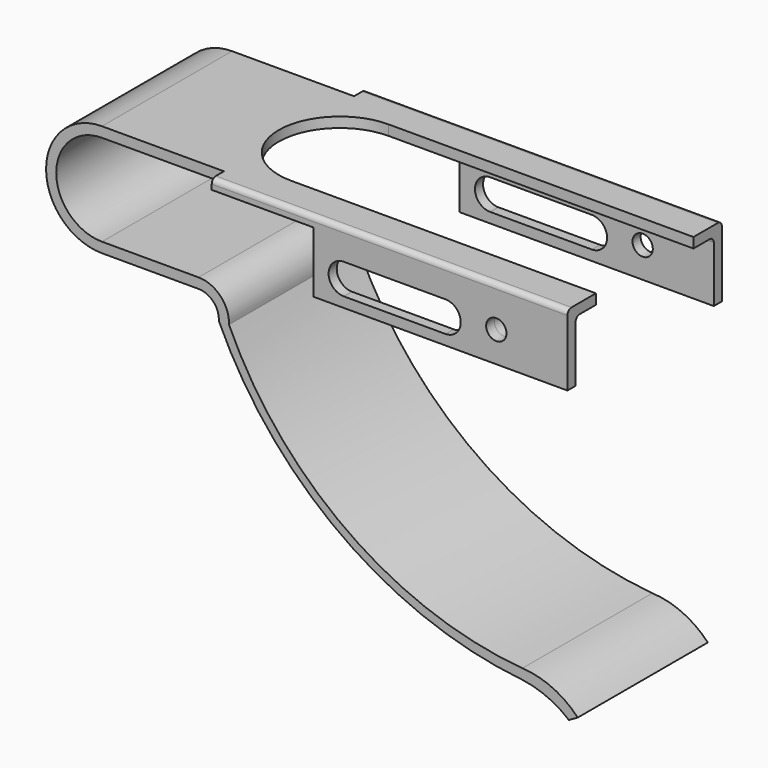
from build123d import *

# Parameters (mm, degrees)
F1_DEPTH  = 16
F2_W      = 70
F2_H      = 3
F3_DEPTH  = 2
F4_W      = 50
F4_H      = 12
F5_DEPTH  = 2
F6_R      = 1
F9_DEPTH  = 2
F11_DEPTH = 38.001
F13_D     = 4
F14_R     = 3
F14_R_2   = 2
F15_DEPTH = 5


with BuildPart() as f1:
    # F0 (on Front) → F1 (new body)
    with BuildSketch(Plane.XZ):
        with BuildLine():
            Line((46.2855722755, 5.7414249778), (-47.7144277245, 5.7414249778))
            ThreePointArc((-47.7144277245, 5.7414249778), (-58.7144277245, -5.2585750222), (-47.7144277245, -16.2585750222))
            Line((-47.7144277245, -16.2585750222), (-28.7144277245, -16.2585750222))
            ThreePointArc((-28.7144277245, -16.2585750222), (-25.7968307423, -17.5210599177), (-24.7197856057, -20.5120821569))
            ThreePointArc((-24.7197856057, -20.5120821569), (-0.5386319719, -49.8206199667), (35.0020481502, -63.2585750222))
            ThreePointArc((35.0020481502, -63.2585750222), (39.8678360266, -64.6074545818), (44.1721712505, -67.2471640366))
            Line((44.1721712505, -67.2471640366), (45.9107602648, -66.2585750222))
            ThreePointArc((45.9107602648, -66.2585750222), (40.9429054682, -62.6971545828), (35.0020481502, -61.2585750222))
            ThreePointArc((35.0020481502, -61.2585750222), (0.6230450398, -48.7022972109), (-22.7197856057, -20.5120821569))
            ThreePointArc((-22.7197856057, -20.5120821569), (-24.3830859689, -16.1065299122), (-28.7144277245, -14.2585750222))
            Line((-28.7144277245, -14.2585750222), (-47.7144277245, -14.2585750222))
            ThreePointArc((-47.7144277245, -14.2585750222), (-56.7144277245, -5.2585750222), (-47.7144277245, 3.7414249778))
            Line((-47.7144277245, 3.7414249778), (46.2855722755, 3.7414249778))
            Line((46.2855722755, 3.7414249778), (46.2855722755, 5.7414249778))
        make_face()
    extrude(amount=F1_DEPTH)

    # F2 (on face) → F3 (join)
    with BuildSketch(Plane.XY.offset(5.7414249778)):
        with Locations((11.2855722755, -17.5)):
            Rectangle(F2_W, F2_H)
    extrude(amount=-F3_DEPTH)

    # F4 (on face) → F5 (join)
    with BuildSketch(Plane.XZ.offset(19)):
        with Locations((21.2855722755, -2.2585750222)):
            Rectangle(F4_W, F4_H)
    extrude(amount=-F5_DEPTH)

    # F6
    f6_edges = [f1.edges().sort_by_distance(p)[0] for p in [
        (11.285572, -19, 5.741425),
        (21.285572, -17, 3.741425),
    ]]
    fillet(f6_edges, radius=F6_R)

    # F7: F1 across plane


with BuildPart() as f1_1:
    add(f1.part)
    add(f1.part.mirror(Plane.XZ))

    # F8 (on face) → F9 (cut)
    with BuildSketch(Plane.XY.offset(5.7414249778)):
        with BuildLine():
            Line((46.2855722755, 12), (-13.7144277245, 12))
            ThreePointArc((-13.7144277245, 12), (-25.7144277245, 0), (-13.7144277245, -12))
            Line((-13.7144277245, -12), (46.2855722755, -12))
            Line((46.2855722755, -12), (46.2855722755, 12))
        make_face()
    extrude(amount=-F9_DEPTH, mode=Mode.SUBTRACT)

    # F10 (on face) → F11 (cut, through all)
    with BuildSketch(Plane.XZ.offset(19)):
        with BuildLine():
            ThreePointArc((2.2855722755, -0.2585750222), (-0.7144277245, -3.2585750222), (2.2855722755, -6.2585750222))
            Line((2.2855722755, -6.2585750222), (22.2855722755, -6.2585750222))
            ThreePointArc((22.2855722755, -6.2585750222), (25.2855722755, -3.2585750222), (22.2855722755, -0.2585750222))
            Line((22.2855722755, -0.2585750222), (2.2855722755, -0.2585750222))
        make_face()
    extrude(amount=-F11_DEPTH, mode=Mode.SUBTRACT)

    # F13 (through all)
    with Locations(Plane.XZ.offset(19)):
        with Locations((32.2855722755, -2.2585750222)):
            Hole(F13_D / 2)

    # F14 (on face) → F15 (join)
    with BuildSketch(Plane(origin=(0, -17, 0), x_dir=(-1, 0, 0), z_dir=(0, 1, 0))):
        with Locations((-32.2855722755, -2.2585750222)):
            Circle(F14_R)
        with Locations((-32.2855722755, -2.2585750222)):
            Circle(F14_R_2, mode=Mode.SUBTRACT)
    extrude(amount=F15_DEPTH)


solid = f1_1.part
